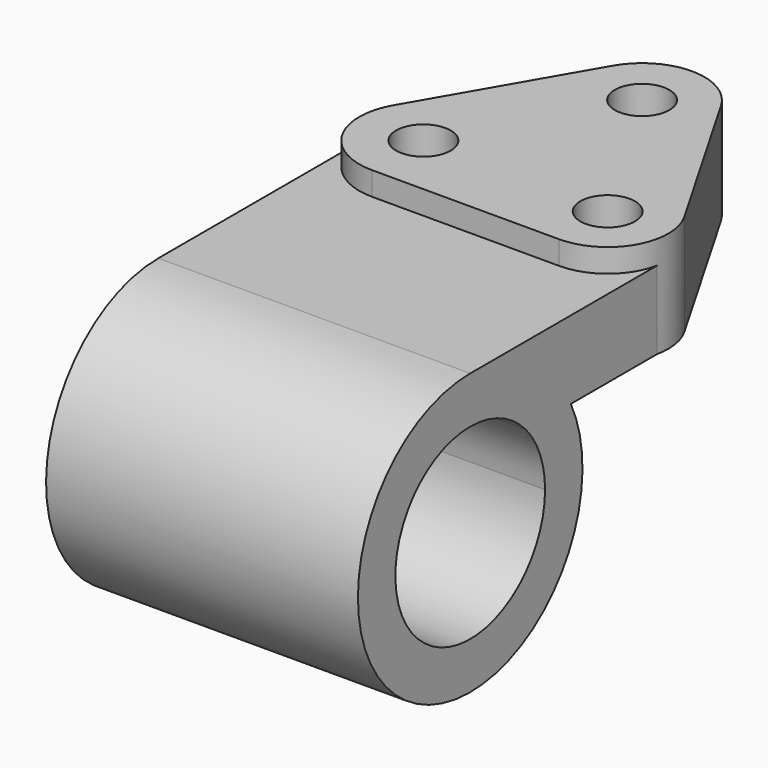
from build123d import *
from build123d import SkipClean  # not in build123d's __all__

# Parameters (mm, degrees)
F0_R          = 5.5626
F1_DEPTH      = 20.6502
F2_W          = 63.5
F2_H          = 15.875
F3_DEPTH      = 37.7444
F3_DEPTH_BACK = 13.0556
F4_R          = 5.5626
F5_DEPTH      = 20.6512
F7_DEPTH      = 63.5
F8_DEPTH      = 63.501
F11_START     = -26.9875
F11_DEPTH     = 9.525


with BuildPart() as f1:
    # F0 (on Top) → F1 (new body)
    with BuildSketch(Plane.XY):
        with BuildLine():
            Line((-18.423879, -23.695093), (19.676121, -23.695093))
            ThreePointArc((19.676121, -23.695093), (30.358613, -17.527553), (30.358613, -5.192474))
            Line((30.358613, -5.192474), (10.998523, 28.340186))
            ThreePointArc((10.998523, 28.340186), (0, 34.690186), (-10.998523, 28.340186))
            Line((-10.998523, 28.340186), (-29.732492, -4.108001))
            ThreePointArc((-29.732492, -4.108001), (-29.732492, -17.166062), (-18.423879, -23.695093))
        make_face()
        with Locations((-18.423879, -10.637032)):
            Circle(F0_R, mode=Mode.SUBTRACT)
        with Locations((19.676121, -11.360014)):
            Circle(F0_R, mode=Mode.SUBTRACT)
        with Locations((0, 21.990186)):
            Circle(F0_R, mode=Mode.SUBTRACT)
    extrude(amount=F1_DEPTH)

    # F2 (on face) → F3 (join, two sides)
    with BuildSketch(Plane.XZ.offset(23.695093)) as f3_sk:
        with Locations((0, 7.9375)):
            Rectangle(F2_W, F2_H)
    extrude(amount=F3_DEPTH)
    extrude(f3_sk.sketch, amount=-F3_DEPTH_BACK)

    # F4 (on face) → F5 (cut, through all)
    with BuildSketch(Plane.XY.offset(20.6502)):
        with Locations((-18.423879, -10.637032)):
            Circle(F4_R)
        with Locations((19.676121, -11.360014)):
            Circle(F4_R)
    extrude(amount=-F5_DEPTH, mode=Mode.SUBTRACT)

    # F6 (on face) → F7 (join, through all)
    with BuildSketch(Plane.YZ.offset(31.75)):
        with BuildLine():
            Line((-61.439493, 6.35), (-61.439493, 15.875))
            ThreePointArc((-61.439493, 15.875), (-76.49984, -36.98408), (-35.841825, 0))
            Line((-35.841825, 0), (-47.240461, 0))
            ThreePointArc((-47.240461, 0), (-43.64351, -5.902539), (-42.389493, -12.7))
            ThreePointArc((-42.389493, -12.7), (-74.909877, -26.170384), (-61.439493, 6.35))
        make_face()
    extrude(amount=-F7_DEPTH)

    # F6 (on face) → F8 (cut, through all)
    with BuildSketch(Plane.YZ.offset(31.75)):
        with BuildLine():
            ThreePointArc((-47.240461, 0), (-53.662363, 4.690191), (-61.439493, 6.35))
            Line((-61.439493, 6.35), (-61.439493, 0))
            Line((-61.439493, 0), (-47.240461, 0))
        make_face()
    with SkipClean():  # cleaning this boolean's faces spoils the solid; the shape is the same uncleaned
        extrude(amount=-F8_DEPTH, mode=Mode.SUBTRACT)

    # F10 (on face) → F11 (join)
    with BuildSketch(Plane.YZ.offset(31.75).offset(F11_START)):
        Polygon((-45.296271, -36.278104), (7.689986, 0), (-35.841825, 0), align=None)
    extrude(amount=-F11_DEPTH)


solid = f1.part
